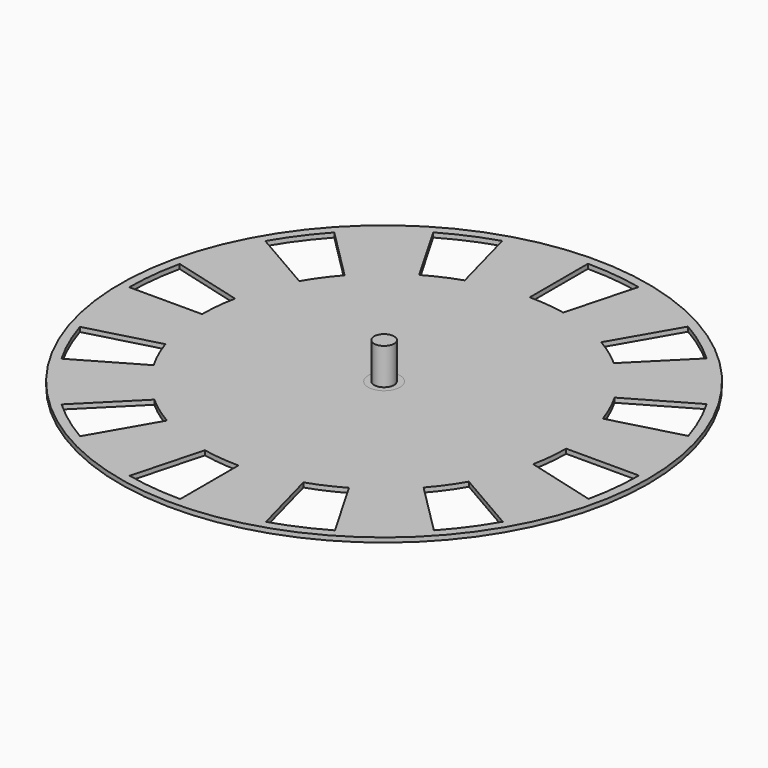
from build123d import *

# Parameters (mm, degrees)
F0_R      = 290
F1_DEPTH  = 5
F2_R      = 11
F3_DEPTH  = 25
F4_DEPTH  = 40
F5_R      = 143.6188138999
F5_R_2    = 11
F6_DEPTH  = 5
F7_R      = 17.5
F7_R_2    = 11
F8_DEPTH  = 25
F9_R      = 17.5
F9_R_2    = 11
F10_DEPTH = 5


with BuildPart() as f1:
    # F0 (on Top) → F1 (new body)
    with BuildSketch(Plane.XY):
        Circle(F0_R)
        with BuildLine():
            Line((-60.9060232783, -273.2955475825), (-40.1742534792, -195.9235293613))
            ThreePointArc((-40.1742534792, -195.9235293613), (-20.1902715155, -198.9782725227), (0, -200))
            Line((0, -200), (0, -280))
            ThreePointArc((0, -280), (-30.6369603331, -278.3188399328), (-60.9060232783, -273.2955475825))
        make_face(mode=Mode.SUBTRACT)
        with BuildLine():
            Line((-189.3939371938, -206.2278753084), (-132.7536887717, -149.5876268864))
            ThreePointArc((-132.7536887717, -149.5876268864), (-116.9744243031, -162.2251030481), (-100, -173.2050807569))
            Line((-100, -173.2050807569), (-140, -242.4871130596))
            ThreePointArc((-140, -242.4871130596), (-165.6918059096, -225.7127055671), (-189.3939371938, -206.2278753084))
        make_face(mode=Mode.SUBTRACT)
        with BuildLine():
            Line((-267.1338985868, -83.9016103887), (-189.7618803656, -63.1698405896))
            ThreePointArc((-189.7618803656, -63.1698405896), (-182.4153745636, -82.0038482196), (-173.2050807569, -100))
            Line((-173.2050807569, -100), (-242.4871130596, -140))
            ThreePointArc((-242.4871130596, -140), (-256.3496659002, -112.6270340232), (-267.1338985868, -83.9016103887))
        make_face(mode=Mode.SUBTRACT)
        with BuildLine():
            Line((-87.8987052892, -104.7543223331), (-73.813275879, -87.9678451288))
            ThreePointArc((-73.813275879, -87.9678451288), (-70.6984313943, -90.4901832852), (-67.4974601638, -92.9022838472))
            Line((-67.4974601638, -92.9022838472), (-80.3776730954, -110.6303760581))
            ThreePointArc((-80.3776730954, -110.6303760581), (-84.1894701397, -107.7579860455), (-87.8987052892, -104.7543223331))
        make_face(mode=Mode.SUBTRACT)
        with BuildLine():
            Line((-103.2037127424, -89.7142358557), (-86.6657147603, -75.337874656))
            ThreePointArc((-86.6657147603, -75.337874656), (-83.9837998001, -78.3164276747), (-81.1995734982, -81.1995734982))
            Line((-81.1995734982, -81.1995734982), (-96.6944942564, -96.6944942564))
            ThreePointArc((-96.6944942564, -96.6944942564), (-100.0100209587, -93.2611716998), (-103.2037127424, -89.7142358557))
        make_face(mode=Mode.SUBTRACT)
        with BuildLine():
            Line((-70.4293399927, -117.215009735), (-59.1433091734, -98.431755306))
            ThreePointArc((-59.1433091734, -98.431755306), (-55.6722329729, -100.4357702634), (-52.1333353489, -102.3174316429))
            Line((-52.1333353489, -102.3174316429), (-62.0816868647, -121.8421708401))
            ThreePointArc((-62.0816868647, -121.8421708401), (-66.295895157, -119.6014411465), (-70.4293399927, -117.215009735))
        make_face(mode=Mode.SUBTRACT)
        with BuildLine():
            Line((-51.225770604, -126.7894745829), (-43.0170379105, -106.4719489913))
            ThreePointArc((-43.0170379105, -106.4719489913), (-39.2751994101, -107.9082952506), (-35.4855147971, -109.2131846994))
            Line((-35.4855147971, -109.2131846994), (-42.257043466, -130.053807005))
            ThreePointArc((-42.257043466, -130.053807005), (-46.7698952121, -128.499911832), (-51.225770604, -126.7894745829))
        make_face(mode=Mode.SUBTRACT)
        with BuildLine():
            Line((-30.7608527345, -133.2419617765), (-25.8315444089, -111.8904499323))
            ThreePointArc((-25.8315444089, -111.8904499323), (-21.911080091, -112.7237598816), (-17.9639231014, -113.4197466908))
            Line((-17.9639231014, -113.4197466908), (-21.3918914141, -135.0630868177))
            ThreePointArc((-21.3918914141, -135.0630868177), (-26.0922652267, -134.2342882215), (-30.7608527345, -133.2419617765))
        make_face(mode=Mode.SUBTRACT)
        with BuildLine():
            Line((-9.5385005812, -136.4135896663), (-8.009992554, -114.5538366528))
            ThreePointArc((-8.009992554, -114.5538366528), (-4.0074372614, -114.7635914356), (0, -114.8335381001))
            Line((0, -114.8335381001), (0, -136.7466651842))
            ThreePointArc((0, -136.7466651842), (-4.7721570762, -136.6633709369), (-9.5385005812, -136.4135896663))
        make_face(mode=Mode.SUBTRACT)
        with BuildLine():
            Line((-125.8757870263, -53.4316074951), (-105.704676351, -44.8693979248))
            ThreePointArc((-105.704676351, -44.8693979248), (-104.0744471533, -48.5309274826), (-102.3174316429, -52.1333353489))
            Line((-102.3174316429, -52.1333353489), (-121.8421708401, -62.0816868647))
            ThreePointArc((-121.8421708401, -62.0816868647), (-123.9344690982, -57.7918489784), (-125.8757870263, -53.4316074951))
        make_face(mode=Mode.SUBTRACT)
        with BuildLine():
            Line((-115.9675022744, -72.4650871471), (-97.3841561172, -60.852835677))
            ThreePointArc((-97.3841561172, -60.852835677), (-95.2012083286, -64.2142616976), (-92.9022838472, -67.4974601638))
            Line((-92.9022838472, -67.4974601638), (-110.6303760581, -80.3776730954))
            ThreePointArc((-110.6303760581, -80.3776730954), (-113.3679931475, -76.4679577908), (-115.9675022744, -72.4650871471))
        make_face(mode=Mode.SUBTRACT)
        with BuildLine():
            Line((-132.6845921438, -33.0824643372), (-111.4223966393, -27.7811266826))
            ThreePointArc((-111.4223966393, -27.7811266826), (-110.3850276859, -31.652600768), (-109.2131846994, -35.4855147971))
            Line((-109.2131846994, -35.4855147971), (-130.053807005, -42.257043466))
            ThreePointArc((-130.053807005, -42.257043466), (-131.4492671047, -37.692713044), (-132.6845921438, -33.0824643372))
        make_face(mode=Mode.SUBTRACT)
        with BuildLine():
            Line((-136.2262622479, -11.9187211129), (-114.3965277326, -10.0087919012))
            ThreePointArc((-114.3965277326, -10.0087919012), (-113.9775624899, -13.9948819736), (-113.4197466908, -17.9639231014))
            Line((-113.4197466908, -17.9639231014), (-135.0630868177, -21.3918914141))
            ThreePointArc((-135.0630868177, -21.3918914141), (-135.7273479001, -16.6654574195), (-136.2262622479, -11.9187211129))
        make_face(mode=Mode.SUBTRACT)
        with BuildLine():
            Line((83.9016103887, -267.1338985868), (63.1698405896, -189.7618803656))
            ThreePointArc((63.1698405896, -189.7618803656), (82.0038482196, -182.4153745636), (100, -173.2050807569))
            Line((100, -173.2050807569), (140, -242.4871130596))
            ThreePointArc((140, -242.4871130596), (112.6270340232, -256.3496659002), (83.9016103887, -267.1338985868))
        make_face(mode=Mode.SUBTRACT)
        with BuildLine():
            Line((11.9187211129, -136.2262622479), (10.0087919012, -114.3965277326))
            ThreePointArc((10.0087919012, -114.3965277326), (13.9948819736, -113.9775624899), (17.9639231014, -113.4197466908))
            Line((17.9639231014, -113.4197466908), (21.3918914141, -135.0630868177))
            ThreePointArc((21.3918914141, -135.0630868177), (16.6654574195, -135.7273479001), (11.9187211129, -136.2262622479))
        make_face(mode=Mode.SUBTRACT)
        with BuildLine():
            Line((33.0824643372, -132.6845921438), (27.7811266826, -111.4223966393))
            ThreePointArc((27.7811266826, -111.4223966393), (31.652600768, -110.3850276859), (35.4855147971, -109.2131846994))
            Line((35.4855147971, -109.2131846994), (42.257043466, -130.053807005))
            ThreePointArc((42.257043466, -130.053807005), (37.692713044, -131.4492671047), (33.0824643372, -132.6845921438))
        make_face(mode=Mode.SUBTRACT)
        with BuildLine():
            Line((53.4316074951, -125.8757870263), (44.8693979248, -105.704676351))
            ThreePointArc((44.8693979248, -105.704676351), (48.5309274826, -104.0744471533), (52.1333353489, -102.3174316429))
            Line((52.1333353489, -102.3174316429), (62.0816868647, -121.8421708401))
            ThreePointArc((62.0816868647, -121.8421708401), (57.7918489784, -123.9344690982), (53.4316074951, -125.8757870263))
        make_face(mode=Mode.SUBTRACT)
        with BuildLine():
            Line((72.4650871471, -115.9675022744), (60.852835677, -97.3841561172))
            ThreePointArc((60.852835677, -97.3841561172), (64.2142616976, -95.2012083286), (67.4974601638, -92.9022838472))
            Line((67.4974601638, -92.9022838472), (80.3776730954, -110.6303760581))
            ThreePointArc((80.3776730954, -110.6303760581), (76.4679577908, -113.3679931475), (72.4650871471, -115.9675022744))
        make_face(mode=Mode.SUBTRACT)
        with BuildLine():
            Line((89.7142358557, -103.2037127424), (75.337874656, -86.6657147603))
            ThreePointArc((75.337874656, -86.6657147603), (78.3164276747, -83.9837998001), (81.1995734982, -81.1995734982))
            Line((81.1995734982, -81.1995734982), (96.6944942564, -96.6944942564))
            ThreePointArc((96.6944942564, -96.6944942564), (93.2611716998, -100.0100209587), (89.7142358557, -103.2037127424))
        make_face(mode=Mode.SUBTRACT)
        with BuildLine():
            Line((104.7543223331, -87.8987052892), (87.9678451288, -73.813275879))
            ThreePointArc((87.9678451288, -73.813275879), (90.4901832852, -70.6984313943), (92.9022838472, -67.4974601638))
            Line((92.9022838472, -67.4974601638), (110.6303760581, -80.3776730954))
            ThreePointArc((110.6303760581, -80.3776730954), (107.7579860455, -84.1894701397), (104.7543223331, -87.8987052892))
        make_face(mode=Mode.SUBTRACT)
        with BuildLine():
            Line((117.215009735, -70.4293399927), (98.431755306, -59.1433091734))
            ThreePointArc((98.431755306, -59.1433091734), (100.4357702634, -55.6722329729), (102.3174316429, -52.1333353489))
            Line((102.3174316429, -52.1333353489), (121.8421708401, -62.0816868647))
            ThreePointArc((121.8421708401, -62.0816868647), (119.6014411465, -66.295895157), (117.215009735, -70.4293399927))
        make_face(mode=Mode.SUBTRACT)
        with BuildLine():
            Line((126.7894745829, -51.225770604), (106.4719489913, -43.0170379105))
            ThreePointArc((106.4719489913, -43.0170379105), (107.9082952506, -39.2751994101), (109.2131846994, -35.4855147971))
            Line((109.2131846994, -35.4855147971), (130.053807005, -42.257043466))
            ThreePointArc((130.053807005, -42.257043466), (128.499911832, -46.7698952121), (126.7894745829, -51.225770604))
        make_face(mode=Mode.SUBTRACT)
        with BuildLine():
            Line((133.2419617765, -30.7608527345), (111.8904499323, -25.8315444089))
            ThreePointArc((111.8904499323, -25.8315444089), (112.7237598816, -21.911080091), (113.4197466908, -17.9639231014))
            Line((113.4197466908, -17.9639231014), (135.0630868177, -21.3918914141))
            ThreePointArc((135.0630868177, -21.3918914141), (134.2342882215, -26.0922652267), (133.2419617765, -30.7608527345))
        make_face(mode=Mode.SUBTRACT)
        with BuildLine():
            Line((136.4135896663, -9.5385005812), (114.5538366528, -8.009992554))
            ThreePointArc((114.5538366528, -8.009992554), (114.7635914356, -4.0074372614), (114.8335381001, 0))
            Line((114.8335381001, 0), (136.7466651842, 0))
            ThreePointArc((136.7466651842, 0), (136.6633709369, -4.7721570762), (136.4135896663, -9.5385005812))
        make_face(mode=Mode.SUBTRACT)
        with BuildLine():
            Line((206.2278753084, -189.3939371938), (149.5876268864, -132.7536887717))
            ThreePointArc((149.5876268864, -132.7536887717), (162.2251030481, -116.9744243031), (173.2050807569, -100))
            Line((173.2050807569, -100), (242.4871130596, -140))
            ThreePointArc((242.4871130596, -140), (225.7127055671, -165.6918059096), (206.2278753084, -189.3939371938))
        make_face(mode=Mode.SUBTRACT)
        with BuildLine():
            Line((273.2955475825, -60.9060232783), (195.9235293613, -40.1742534792))
            ThreePointArc((195.9235293613, -40.1742534792), (198.9782725227, -20.1902715155), (200, 0))
            Line((200, 0), (280, 0))
            ThreePointArc((280, 0), (278.3188399328, -30.6369603331), (273.2955475825, -60.9060232783))
        make_face(mode=Mode.SUBTRACT)
        with BuildLine():
            Line((-273.2955475825, 60.9060232783), (-195.9235293613, 40.1742534792))
            ThreePointArc((-195.9235293613, 40.1742534792), (-198.9782725227, 20.1902715155), (-200, 0))
            Line((-200, 0), (-280, 0))
            ThreePointArc((-280, 0), (-278.3188399328, 30.6369603331), (-273.2955475825, 60.9060232783))
        make_face(mode=Mode.SUBTRACT)
        with BuildLine():
            Line((-206.2278753084, 189.3939371938), (-149.5876268864, 132.7536887717))
            ThreePointArc((-149.5876268864, 132.7536887717), (-162.2251030481, 116.9744243031), (-173.2050807569, 100))
            Line((-173.2050807569, 100), (-242.4871130596, 140))
            ThreePointArc((-242.4871130596, 140), (-225.7127055671, 165.6918059096), (-206.2278753084, 189.3939371938))
        make_face(mode=Mode.SUBTRACT)
        with BuildLine():
            Line((-136.4135896663, 9.5385005812), (-114.5538366528, 8.009992554))
            ThreePointArc((-114.5538366528, 8.009992554), (-114.7635914356, 4.0074372614), (-114.8335381001, 0))
            Line((-114.8335381001, 0), (-136.7466651842, 0))
            ThreePointArc((-136.7466651842, 0), (-136.6633709369, 4.7721570762), (-136.4135896663, 9.5385005812))
        make_face(mode=Mode.SUBTRACT)
        with BuildLine():
            Line((-133.2419617765, 30.7608527345), (-111.8904499323, 25.8315444089))
            ThreePointArc((-111.8904499323, 25.8315444089), (-112.7237598816, 21.911080091), (-113.4197466908, 17.9639231014))
            Line((-113.4197466908, 17.9639231014), (-135.0630868177, 21.3918914141))
            ThreePointArc((-135.0630868177, 21.3918914141), (-134.2342882215, 26.0922652267), (-133.2419617765, 30.7608527345))
        make_face(mode=Mode.SUBTRACT)
        with BuildLine():
            Line((-126.7894745829, 51.225770604), (-106.4719489913, 43.0170379105))
            ThreePointArc((-106.4719489913, 43.0170379105), (-107.9082952506, 39.2751994101), (-109.2131846994, 35.4855147971))
            Line((-109.2131846994, 35.4855147971), (-130.053807005, 42.257043466))
            ThreePointArc((-130.053807005, 42.257043466), (-128.499911832, 46.7698952121), (-126.7894745829, 51.225770604))
        make_face(mode=Mode.SUBTRACT)
        with BuildLine():
            Line((-117.215009735, 70.4293399927), (-98.431755306, 59.1433091734))
            ThreePointArc((-98.431755306, 59.1433091734), (-100.4357702634, 55.6722329729), (-102.3174316429, 52.1333353489))
            Line((-102.3174316429, 52.1333353489), (-121.8421708401, 62.0816868647))
            ThreePointArc((-121.8421708401, 62.0816868647), (-119.6014411465, 66.295895157), (-117.215009735, 70.4293399927))
        make_face(mode=Mode.SUBTRACT)
        with BuildLine():
            Line((-104.7543223331, 87.8987052892), (-87.9678451288, 73.813275879))
            ThreePointArc((-87.9678451288, 73.813275879), (-90.4901832852, 70.6984313943), (-92.9022838472, 67.4974601638))
            Line((-92.9022838472, 67.4974601638), (-110.6303760581, 80.3776730954))
            ThreePointArc((-110.6303760581, 80.3776730954), (-107.7579860455, 84.1894701397), (-104.7543223331, 87.8987052892))
        make_face(mode=Mode.SUBTRACT)
        with BuildLine():
            Line((-89.7142358557, 103.2037127424), (-75.337874656, 86.6657147603))
            ThreePointArc((-75.337874656, 86.6657147603), (-78.3164276747, 83.9837998001), (-81.1995734982, 81.1995734982))
            Line((-81.1995734982, 81.1995734982), (-96.6944942564, 96.6944942564))
            ThreePointArc((-96.6944942564, 96.6944942564), (-93.2611716998, 100.0100209587), (-89.7142358557, 103.2037127424))
        make_face(mode=Mode.SUBTRACT)
        with BuildLine():
            Line((-72.4650871471, 115.9675022744), (-60.852835677, 97.3841561172))
            ThreePointArc((-60.852835677, 97.3841561172), (-64.2142616976, 95.2012083286), (-67.4974601638, 92.9022838472))
            Line((-67.4974601638, 92.9022838472), (-80.3776730954, 110.6303760581))
            ThreePointArc((-80.3776730954, 110.6303760581), (-76.4679577908, 113.3679931475), (-72.4650871471, 115.9675022744))
        make_face(mode=Mode.SUBTRACT)
        with BuildLine():
            Line((-53.4316074951, 125.8757870263), (-44.8693979248, 105.704676351))
            ThreePointArc((-44.8693979248, 105.704676351), (-48.5309274826, 104.0744471533), (-52.1333353489, 102.3174316429))
            Line((-52.1333353489, 102.3174316429), (-62.0816868647, 121.8421708401))
            ThreePointArc((-62.0816868647, 121.8421708401), (-57.7918489784, 123.9344690982), (-53.4316074951, 125.8757870263))
        make_face(mode=Mode.SUBTRACT)
        with BuildLine():
            Line((-33.0824643372, 132.6845921438), (-27.7811266826, 111.4223966393))
            ThreePointArc((-27.7811266826, 111.4223966393), (-31.652600768, 110.3850276859), (-35.4855147971, 109.2131846994))
            Line((-35.4855147971, 109.2131846994), (-42.257043466, 130.053807005))
            ThreePointArc((-42.257043466, 130.053807005), (-37.692713044, 131.4492671047), (-33.0824643372, 132.6845921438))
        make_face(mode=Mode.SUBTRACT)
        with BuildLine():
            Line((-11.9187211129, 136.2262622479), (-10.0087919012, 114.3965277326))
            ThreePointArc((-10.0087919012, 114.3965277326), (-13.9948819736, 113.9775624899), (-17.9639231014, 113.4197466908))
            Line((-17.9639231014, 113.4197466908), (-21.3918914141, 135.0630868177))
            ThreePointArc((-21.3918914141, 135.0630868177), (-16.6654574195, 135.7273479001), (-11.9187211129, 136.2262622479))
        make_face(mode=Mode.SUBTRACT)
        with BuildLine():
            Line((-83.9016103887, 267.1338985868), (-63.1698405896, 189.7618803656))
            ThreePointArc((-63.1698405896, 189.7618803656), (-82.0038482196, 182.4153745636), (-100, 173.2050807569))
            Line((-100, 173.2050807569), (-140, 242.4871130596))
            ThreePointArc((-140, 242.4871130596), (-112.6270340232, 256.3496659002), (-83.9016103887, 267.1338985868))
        make_face(mode=Mode.SUBTRACT)
        Polygon((5, 5), (5, -5), (-5, -5), (-5, 5), (0, 5), align=None, mode=Mode.SUBTRACT)
        with BuildLine():
            Line((136.2262622479, 11.9187211129), (114.3965277326, 10.0087919012))
            ThreePointArc((114.3965277326, 10.0087919012), (113.9775624899, 13.9948819736), (113.4197466908, 17.9639231014))
            Line((113.4197466908, 17.9639231014), (135.0630868177, 21.3918914141))
            ThreePointArc((135.0630868177, 21.3918914141), (135.7273479001, 16.6654574195), (136.2262622479, 11.9187211129))
        make_face(mode=Mode.SUBTRACT)
        with BuildLine():
            Line((132.6845921438, 33.0824643372), (111.4223966393, 27.7811266826))
            ThreePointArc((111.4223966393, 27.7811266826), (110.3850276859, 31.652600768), (109.2131846994, 35.4855147971))
            Line((109.2131846994, 35.4855147971), (130.053807005, 42.257043466))
            ThreePointArc((130.053807005, 42.257043466), (131.4492671047, 37.692713044), (132.6845921438, 33.0824643372))
        make_face(mode=Mode.SUBTRACT)
        with BuildLine():
            Line((115.9675022744, 72.4650871471), (97.3841561172, 60.852835677))
            ThreePointArc((97.3841561172, 60.852835677), (95.2012083286, 64.2142616976), (92.9022838472, 67.4974601638))
            Line((92.9022838472, 67.4974601638), (110.6303760581, 80.3776730954))
            ThreePointArc((110.6303760581, 80.3776730954), (113.3679931475, 76.4679577908), (115.9675022744, 72.4650871471))
        make_face(mode=Mode.SUBTRACT)
        with BuildLine():
            Line((125.8757870263, 53.4316074951), (105.704676351, 44.8693979248))
            ThreePointArc((105.704676351, 44.8693979248), (104.0744471533, 48.5309274826), (102.3174316429, 52.1333353489))
            Line((102.3174316429, 52.1333353489), (121.8421708401, 62.0816868647))
            ThreePointArc((121.8421708401, 62.0816868647), (123.9344690982, 57.7918489784), (125.8757870263, 53.4316074951))
        make_face(mode=Mode.SUBTRACT)
        with BuildLine():
            ThreePointArc((0, 136.7466651842), (4.7721570762, 136.6633709369), (9.5385005812, 136.4135896663))
            Line((9.5385005812, 136.4135896663), (8.009992554, 114.5538366528))
            ThreePointArc((8.009992554, 114.5538366528), (4.0074372614, 114.7635914356), (0, 114.8335381001))
            Line((0, 114.8335381001), (0, 136.7466651842))
        make_face(mode=Mode.SUBTRACT)
        with BuildLine():
            Line((30.7608527345, 133.2419617765), (25.8315444089, 111.8904499323))
            ThreePointArc((25.8315444089, 111.8904499323), (21.911080091, 112.7237598816), (17.9639231014, 113.4197466908))
            Line((17.9639231014, 113.4197466908), (21.3918914141, 135.0630868177))
            ThreePointArc((21.3918914141, 135.0630868177), (26.0922652267, 134.2342882215), (30.7608527345, 133.2419617765))
        make_face(mode=Mode.SUBTRACT)
        with BuildLine():
            Line((51.225770604, 126.7894745829), (43.0170379105, 106.4719489913))
            ThreePointArc((43.0170379105, 106.4719489913), (39.2751994101, 107.9082952506), (35.4855147971, 109.2131846994))
            Line((35.4855147971, 109.2131846994), (42.257043466, 130.053807005))
            ThreePointArc((42.257043466, 130.053807005), (46.7698952121, 128.499911832), (51.225770604, 126.7894745829))
        make_face(mode=Mode.SUBTRACT)
        with BuildLine():
            Line((70.4293399927, 117.215009735), (59.1433091734, 98.431755306))
            ThreePointArc((59.1433091734, 98.431755306), (55.6722329729, 100.4357702634), (52.1333353489, 102.3174316429))
            Line((52.1333353489, 102.3174316429), (62.0816868647, 121.8421708401))
            ThreePointArc((62.0816868647, 121.8421708401), (66.295895157, 119.6014411465), (70.4293399927, 117.215009735))
        make_face(mode=Mode.SUBTRACT)
        with BuildLine():
            Line((103.2037127424, 89.7142358557), (86.6657147603, 75.337874656))
            ThreePointArc((86.6657147603, 75.337874656), (83.9837998001, 78.3164276747), (81.1995734982, 81.1995734982))
            Line((81.1995734982, 81.1995734982), (96.6944942564, 96.6944942564))
            ThreePointArc((96.6944942564, 96.6944942564), (100.0100209587, 93.2611716998), (103.2037127424, 89.7142358557))
        make_face(mode=Mode.SUBTRACT)
        with BuildLine():
            Line((87.8987052892, 104.7543223331), (73.813275879, 87.9678451288))
            ThreePointArc((73.813275879, 87.9678451288), (70.6984313943, 90.4901832852), (67.4974601638, 92.9022838472))
            Line((67.4974601638, 92.9022838472), (80.3776730954, 110.6303760581))
            ThreePointArc((80.3776730954, 110.6303760581), (84.1894701397, 107.7579860455), (87.8987052892, 104.7543223331))
        make_face(mode=Mode.SUBTRACT)
        with BuildLine():
            Line((267.1338985868, 83.9016103887), (189.7618803656, 63.1698405896))
            ThreePointArc((189.7618803656, 63.1698405896), (182.4153745636, 82.0038482196), (173.2050807569, 100))
            Line((173.2050807569, 100), (242.4871130596, 140))
            ThreePointArc((242.4871130596, 140), (256.3496659002, 112.6270340232), (267.1338985868, 83.9016103887))
        make_face(mode=Mode.SUBTRACT)
        with BuildLine():
            Line((189.3939371938, 206.2278753084), (132.7536887717, 149.5876268864))
            ThreePointArc((132.7536887717, 149.5876268864), (116.9744243031, 162.2251030481), (100, 173.2050807569))
            Line((100, 173.2050807569), (140, 242.4871130596))
            ThreePointArc((140, 242.4871130596), (165.6918059096, 225.7127055671), (189.3939371938, 206.2278753084))
        make_face(mode=Mode.SUBTRACT)
        with BuildLine():
            Line((60.9060232783, 273.2955475825), (40.1742534792, 195.9235293613))
            ThreePointArc((40.1742534792, 195.9235293613), (20.1902715155, 198.9782725227), (0, 200))
            Line((0, 200), (0, 280))
            ThreePointArc((0, 280), (30.6369603331, 278.3188399328), (60.9060232783, 273.2955475825))
        make_face(mode=Mode.SUBTRACT)
    extrude(amount=F1_DEPTH)

    # F2 (on face) → F3 (cut)
    with BuildSketch(Plane.XY.offset(5)):
        Circle(F2_R)
    extrude(amount=-F3_DEPTH, mode=Mode.SUBTRACT)



with BuildPart() as f4:
    # F2 (on face) → F4 (new body, symmetric)
    with BuildSketch(Plane.XY.offset(5)):
        Circle(F2_R)
    extrude(amount=F4_DEPTH, both=True)


with BuildPart() as f1_1:
    add(f1.part)

    add(f4.part)  # F6 merges F4
    # F5 (on face) → F6 (join)
    with BuildSketch(Plane.XY.offset(5)):
        Circle(F5_R)
        Circle(F5_R_2, mode=Mode.SUBTRACT)
    extrude(amount=-F6_DEPTH)

    # F7 (on face) → F8 (cut)
    with BuildSketch(Plane.XY.offset(5)):
        Circle(F7_R)
        Circle(F7_R_2, mode=Mode.SUBTRACT)
    extrude(amount=-F8_DEPTH, mode=Mode.SUBTRACT)


with BuildPart() as f10:
    # F9 (on face) → F10 (new body)
    with BuildSketch(Plane.XY.offset(5)):
        Circle(F9_R)
        Circle(F9_R_2, mode=Mode.SUBTRACT)
    extrude(amount=-F10_DEPTH)


solid = Compound([f1_1.part, f10.part])
